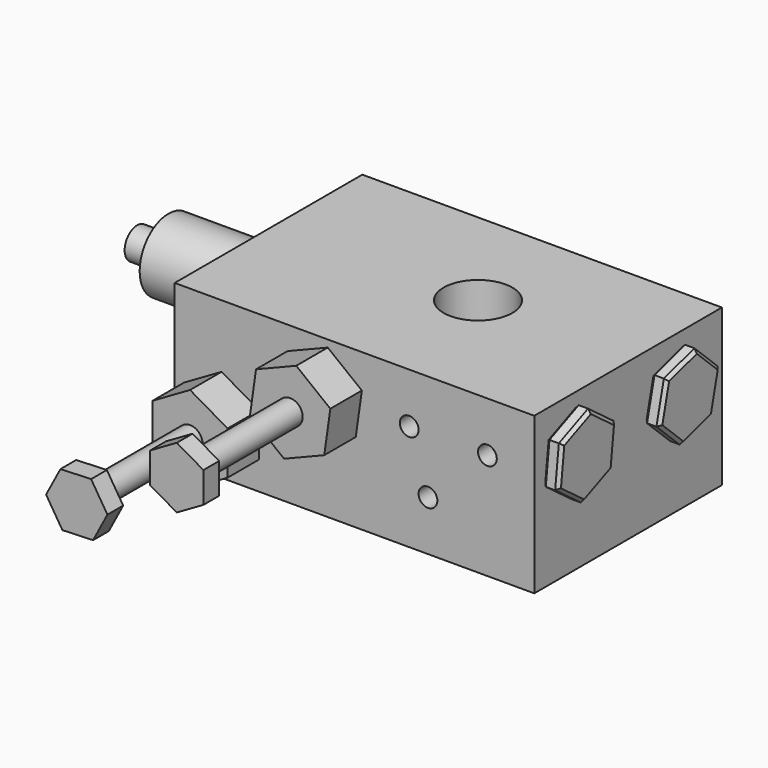
from build123d import *

# Parameters (mm, degrees)
F0_W            = 115
F0_H            = 75
F1_DEPTH        = 50
F3_D            = 5
F3_DEPTH        = 35
F3_TIP          = 1.5021515476
F6_D            = 13
F6_DEPTH        = 27
F6_CBORE_D      = 19
F6_CBORE_DEPTH  = 20
F6_TIP          = 3.9055940237
F8_D            = 6
F8_DEPTH        = 57
F8_TIP          = 1.8025818571
F10_D           = 6
F10_DEPTH       = 83
F10_TIP         = 1.8025818571
F11_D           = 13
F11_DEPTH       = 30
F11_CBORE_D     = 19
F11_CBORE_DEPTH = 22
F11_TIP         = 3.9055940237
F12_D           = 6
F12_DEPTH       = 4
F12_START       = 32.1030122
F12_TIP         = 1.8025818571
F13_D           = 6
F13_DEPTH       = 15
F13_START       = 29.1030122
F13_TIP         = 1.8025818571
F14_D           = 6
F14_DEPTH       = 16
F14_TIP         = 1.8025818571
F15_D           = 6
F15_DEPTH       = 30
F15_START       = 29.1030122
F15_TIP         = 1.8025818571
F16_D           = 6
F16_DEPTH       = 50
F16_TIP         = 1.8025818571
F17_D           = 6
F17_DEPTH       = 34
F17_TIP         = 1.8025818571
F18_D           = 13
F18_DEPTH       = 30
F18_CBORE_D     = 19
F18_CBORE_DEPTH = 22
F18_TIP         = 3.9055940237
F19_D           = 13
F19_DEPTH       = 30
F19_CBORE_D     = 19
F19_CBORE_DEPTH = 22
F19_TIP         = 3.9055940237
F20_D           = 6
F20_DEPTH       = 15
F20_START       = 32.1030122
F20_TIP         = 1.8025818571
F21_D           = 6
F21_DEPTH       = 35
F21_TIP         = 1.8025818571
F22_D           = 6
F22_DEPTH       = 4
F22_START       = 38
F22_TIP         = 1.8025818571
F24_D           = 5
F24_DEPTH       = 15
F24_TIP         = 1.5021515476
F25_D           = 22
F26_R           = 11.5
F27_DEPTH       = 26
F29_D           = 6
F29_DEPTH       = 82
F29_TIP         = 1.8025818571
F30_DEPTH       = 5
F31_SIZE        = 1
F31_2_SIZE      = 1
F28_R           = 5
F32_DEPTH       = 12
F9_R            = 11.5
F33_DEPTH       = 30
F34_R           = 5
F35_DEPTH       = 10
F36_D           = 6
F36_DEPTH       = 18
F36_TIP         = 1.8025818571
F38_DEPTH       = 12.6
F39_R           = 4
F40_DEPTH       = 39
F41_R           = 4
F42_DEPTH       = 6.3
F43_R           = 4
F44_DEPTH       = 39
F45_R           = 4
F46_DEPTH       = 6.3
F47_D           = 5
F47_DEPTH       = 6
F47_TIP         = 1.5021515476


# Not quite as in the source:
# - a feature names something its author has since deleted; it is built from what else it names


with BuildPart() as f1:
    # F0 (on Top) → F1 (new body)
    with BuildSketch(Plane.XY):
        with Locations((-7.5, -2.5)):
            Rectangle(F0_W, F0_H)
    extrude(amount=F1_DEPTH)

    # F3
    with Locations(Plane(origin=(0, 0, 0), x_dir=(1, 0, 0), z_dir=(0, 0, -1))):
        with Locations((-16, -7.32)):
            Hole(F3_D / 2, depth=F3_DEPTH)
            with Locations((0, 0, -(F3_DEPTH + F3_TIP / 2))):  # 118° drill point
                Cone(0, F3_D / 2, F3_TIP, mode=Mode.SUBTRACT)

    # F6
    with Locations(Plane.YZ.offset(50)):
        with Locations((16, 34), (-25, 34)):
            CounterBoreHole(F6_D / 2, F6_CBORE_D / 2, F6_CBORE_DEPTH, depth=F6_DEPTH)
            with Locations((0, 0, -(F6_DEPTH + F6_TIP / 2))):  # 118° drill point
                Cone(0, F6_D / 2, F6_TIP, mode=Mode.SUBTRACT)

    # F8
    with Locations(Plane.XZ.offset(40)):
        with Locations((16, 16)):
            Hole(F8_D / 2, depth=F8_DEPTH)
            with Locations((0, 0, -(F8_DEPTH + F8_TIP / 2))):  # 118° drill point
                Cone(0, F8_D / 2, F8_TIP, mode=Mode.SUBTRACT)

    # F10
    with Locations(Plane(origin=(-65, 0, 0), x_dir=(0, -1, 0), z_dir=(-1, 0, 0))):
        with Locations((25, 16)):
            Hole(F10_D / 2, depth=F10_DEPTH)
            with Locations((0, 0, -(F10_DEPTH + F10_TIP / 2))):  # 118° drill point
                Cone(0, F10_D / 2, F10_TIP, mode=Mode.SUBTRACT)

    # F11
    with Locations(Plane.XZ.offset(40)):
        with Locations((-50, 16), (-18, 34)):
            CounterBoreHole(F11_D / 2, F11_CBORE_D / 2, F11_CBORE_DEPTH, depth=F11_DEPTH)
            with Locations((0, 0, -(F11_DEPTH + F11_TIP / 2))):  # 118° drill point
                Cone(0, F11_D / 2, F11_TIP, mode=Mode.SUBTRACT)

    # F12
    # its depths count from where the whole tool has entered the part; down to there all is cleared
    with Locations(Plane.XZ.offset(40)):
        with Locations((-50, 16)):
            Hole(F12_D / 2, depth=F12_START)
    with Locations(Plane.XZ.offset(40).offset(-F12_START)):
        with Locations((-50, 16)):
            Hole(F12_D / 2, depth=F12_DEPTH)
            with Locations((0, 0, -(F12_DEPTH + F12_TIP / 2))):  # 118° drill point
                Cone(0, F12_D / 2, F12_TIP, mode=Mode.SUBTRACT)

    # F13
    # its depths count from where the whole tool has entered the part; down to there all is cleared
    with Locations(Plane.YZ.offset(50)):
        with Locations((16, 34)):
            Hole(F13_D / 2, depth=F13_START)
    with Locations(Plane.YZ.offset(50).offset(-F13_START)):
        with Locations((16, 34)):
            Hole(F13_D / 2, depth=F13_DEPTH)
            with Locations((0, 0, -(F13_DEPTH + F13_TIP / 2))):  # 118° drill point
                Cone(0, F13_D / 2, F13_TIP, mode=Mode.SUBTRACT)

    # F14
    with Locations(Plane.XZ.offset(40)):
        with Locations((10, 34)):
            Hole(F14_D / 2, depth=F14_DEPTH)
            with Locations((0, 0, -(F14_DEPTH + F14_TIP / 2))):  # 118° drill point
                Cone(0, F14_D / 2, F14_TIP, mode=Mode.SUBTRACT)

    # F15
    # its depths count from where the whole tool has entered the part; down to there all is cleared
    with Locations(Plane.YZ.offset(50).offset(-F15_START)):
        with Locations((-25, 34)):
            Hole(F15_D / 2, depth=F15_DEPTH)
            with Locations((0, 0, -(F15_DEPTH + F15_TIP / 2))):  # 118° drill point
                Cone(0, F15_D / 2, F15_TIP, mode=Mode.SUBTRACT)

    # F16
    with Locations(Plane.XZ.offset(40)):
        with Locations((35, 34)):
            Hole(F16_D / 2, depth=F16_DEPTH)
            with Locations((0, 0, -(F16_DEPTH + F16_TIP / 2))):  # 118° drill point
                Cone(0, F16_D / 2, F16_TIP, mode=Mode.SUBTRACT)

    # F17
    with Locations(Plane(origin=(0, 0, 0), x_dir=(1, 0, 0), z_dir=(0, 0, -1))):
        with Locations((35, 7)):
            Hole(F17_D / 2, depth=F17_DEPTH)
            with Locations((0, 0, -(F17_DEPTH + F17_TIP / 2))):  # 118° drill point
                Cone(0, F17_D / 2, F17_TIP, mode=Mode.SUBTRACT)

    # F18
    with Locations(Plane(origin=(-65, 0, 0), x_dir=(0, -1, 0), z_dir=(-1, 0, 0))):
        with Locations((5, 34)):
            CounterBoreHole(F18_D / 2, F18_CBORE_D / 2, F18_CBORE_DEPTH, depth=F18_DEPTH)
            with Locations((0, 0, -(F18_DEPTH + F18_TIP / 2))):  # 118° drill point
                Cone(0, F18_D / 2, F18_TIP, mode=Mode.SUBTRACT)

    # F19
    with Locations(Plane(origin=(-65, 0, 0), x_dir=(0, -1, 0), z_dir=(-1, 0, 0))):
        with Locations((-16, 16)):
            CounterBoreHole(F19_D / 2, F19_CBORE_D / 2, F19_CBORE_DEPTH, depth=F19_DEPTH)
            with Locations((0, 0, -(F19_DEPTH + F19_TIP / 2))):  # 118° drill point
                Cone(0, F19_D / 2, F19_TIP, mode=Mode.SUBTRACT)

    # F20
    # its depths count from where the whole tool has entered the part; down to there all is cleared
    with Locations(Plane(origin=(-65, 0, 0), x_dir=(0, -1, 0), z_dir=(-1, 0, 0))):
        with Locations((5, 34)):
            Hole(F20_D / 2, depth=F20_START)
    with Locations(Plane(origin=(-65, 0, 0), x_dir=(0, -1, 0), z_dir=(-1, 0, 0)).offset(-F20_START)):
        with Locations((5, 34)):
            Hole(F20_D / 2, depth=F20_DEPTH)
            with Locations((0, 0, -(F20_DEPTH + F20_TIP / 2))):  # 118° drill point
                Cone(0, F20_D / 2, F20_TIP, mode=Mode.SUBTRACT)

    # F21
    with Locations(Plane(origin=(0, 0, 0), x_dir=(1, 0, 0), z_dir=(0, 0, -1))):
        with Locations((-50, 5)):
            Hole(F21_D / 2, depth=F21_DEPTH)
            with Locations((0, 0, -(F21_DEPTH + F21_TIP / 2))):  # 118° drill point
                Cone(0, F21_D / 2, F21_TIP, mode=Mode.SUBTRACT)

    # F22
    # its depths count from where the whole tool has entered the part; down to there all is cleared
    with Locations(Plane.XZ.offset(40)):
        with Locations((-18, 34)):
            Hole(F22_D / 2, depth=F22_START)
    with Locations(Plane.XZ.offset(40).offset(-F22_START)):
        with Locations((-18, 34)):
            Hole(F22_D / 2, depth=F22_DEPTH)
            with Locations((0, 0, -(F22_DEPTH + F22_TIP / 2))):  # 118° drill point
                Cone(0, F22_D / 2, F22_TIP, mode=Mode.SUBTRACT)

    # F24
    with Locations(Plane(origin=(0, 35, 0), x_dir=(-1, 0, 0), z_dir=(0, 1, 0))):
        with Locations((35, 25), (-25, 25)):
            Hole(F24_D / 2, depth=F24_DEPTH)
            with Locations((0, 0, -(F24_DEPTH + F24_TIP / 2))):  # 118° drill point
                Cone(0, F24_D / 2, F24_TIP, mode=Mode.SUBTRACT)

    # F25 (through all)
    with Locations(Plane(origin=(0, 0, 0), x_dir=(1, 0, 0), z_dir=(0, 0, -1))):
        with Locations((0, 0)):
            Hole(F25_D / 2)

    # F29
    with Locations(Plane(origin=(-65, 0, 0), x_dir=(0, -1, 0), z_dir=(-1, 0, 0))):
        with Locations((-16, 16)):
            Hole(F29_D / 2, depth=F29_DEPTH)
            with Locations((0, 0, -(F29_DEPTH + F29_TIP / 2))):  # 118° drill point
                Cone(0, F29_D / 2, F29_TIP, mode=Mode.SUBTRACT)

    # F36
    with Locations(Plane(origin=(0, 0, 0), x_dir=(1, 0, 0), z_dir=(0, 0, -1))):
        with Locations((-50, -16)):
            Hole(F36_D / 2, depth=F36_DEPTH)
            with Locations((0, 0, -(F36_DEPTH + F36_TIP / 2))):  # 118° drill point
                Cone(0, F36_D / 2, F36_TIP, mode=Mode.SUBTRACT)

    # F47
    with Locations(Plane(origin=(0, 0, 0), x_dir=(1, 0, 0), z_dir=(0, 0, -1))):
        with Locations((16, -22.32), (-16, 7.68)):
            Hole(F47_D / 2, depth=F47_DEPTH)
            with Locations((0, 0, -(F47_DEPTH + F47_TIP / 2))):  # 118° drill point
                Cone(0, F47_D / 2, F47_TIP, mode=Mode.SUBTRACT)


with BuildPart() as f27:
    # F26 (on face) → F27 (new body)
    with BuildSketch(Plane(origin=(-65, 0, 0), x_dir=(0, -1, 0), z_dir=(-1, 0, 0))):
        with Locations((-16, 16)):
            Circle(F26_R)
    extrude(amount=F27_DEPTH)

    # F28 (on face) → F32 (join)
    with BuildSketch(Plane(origin=(-91, 0, 0), x_dir=(0, -1, 0), z_dir=(-1, 0, 0))):
        with Locations((-16, 16)):
            Circle(F28_R)
    extrude(amount=F32_DEPTH)


with BuildPart() as f30:
    # F5 (on face) → F30 (new body)
    with BuildSketch(Plane.YZ.offset(50)):
        Polygon((-23.5270221617, 46.6160084663), (-35.189294907, 41.5836404603), (-36.6622727453, 28.967631994), (-26.4729778383, 21.3839915337), (-14.810705093, 26.4163595397), (-13.3377272547, 39.032368006), align=None)
    extrude(amount=F30_DEPTH)

    # F31
    f31_edges = [f30.edges().sort_by_distance(p)[0] for p in [
        (50, -20.641841, 23.900176),
        (50, -31.567625, 25.175812),
        (50, -35.925784, 35.275636),
        (55, -31.567625, 25.175812),
        (55, -20.641841, 23.900176),
        (55, -14.074216, 32.724364),
        (55, -18.432375, 42.824188),
        (55, -29.358159, 44.099824),
        (55, -35.925784, 35.275636),
        (50, -29.358159, 44.099824),
        (50, -18.432375, 42.824188),
        (50, -14.074216, 32.724364),
    ]]
    chamfer(f31_edges, length=F31_SIZE)


with BuildPart() as f30b:
    # F5 (on face) → F30, piece 2 (new body)
    with BuildSketch(Plane.YZ.offset(50)):
        Polygon((18.9808178574, 46.3469857955), (6.7976055696, 42.7549568863), (3.8167877122, 30.4079710908), (13.0191821426, 21.6530142045), (25.2023944304, 25.2450431137), (28.1832122878, 37.5920289092), align=None)
    extrude(amount=F30_DEPTH)

    # F31#2
    f31_2_edges = [f30b.edges().sort_by_distance(p)[0] for p in [
        (55, 8.417985, 26.030493),
        (50, 8.417985, 26.030493),
        (55, 19.110788, 23.449029),
        (50, 19.110788, 23.449029),
        (55, 26.692803, 31.418536),
        (50, 26.692803, 31.418536),
        (55, 23.582015, 41.969507),
        (50, 23.582015, 41.969507),
        (55, 5.307197, 36.581464),
        (50, 5.307197, 36.581464),
        (50, 12.889212, 44.550971),
        (55, 12.889212, 44.550971),
    ]]
    chamfer(f31_2_edges, length=F31_2_SIZE)


with BuildPart() as f33:
    # F9 (on face) → F33 (new body)
    with BuildSketch(Plane(origin=(-65, 0, 0), x_dir=(0, -1, 0), z_dir=(-1, 0, 0))):
        with Locations((5, 34)):
            Circle(F9_R)
    extrude(amount=F33_DEPTH)

    # F34 (on face) → F35 (join)
    with BuildSketch(Plane(origin=(-95, 0, 0), x_dir=(0, -1, 0), z_dir=(-1, 0, 0))):
        with Locations((5, 34)):
            Circle(F34_R)
    extrude(amount=F35_DEPTH)


with BuildPart() as f38:
    # F37 (on face) → F38 (new body)
    with BuildSketch(Plane.XZ.offset(40)):
        Polygon((-38, 9.0717967697), (-38, 22.9282032303), (-50, 29.8564064606), (-62, 22.9282032303), (-62, 9.0717967697), (-50, 2.1435935394), align=None)
    extrude(amount=F38_DEPTH)

    # F39 (on face) → F40 (join)
    with BuildSketch(Plane.XZ.offset(52.6)):
        with Locations((-50, 16)):
            Circle(F39_R)
    extrude(amount=F40_DEPTH)

    # F41 (on face) → F42 (join)
    with BuildSketch(Plane.XZ.offset(91.6)):
        Polygon((-40.1919154978, 16.3671671712), (-45.4139338466, 24.6776339269), (-55.2220183487, 24.3104667558), (-59.8080845022, 15.6328328288), (-54.5860661534, 7.3223660731), (-44.7779816513, 7.6895332442), align=None)
        with Locations((-50, 16)):
            Circle(F41_R, mode=Mode.SUBTRACT)
        with Locations((-50, 16)):
            Circle(F41_R)
    extrude(amount=F42_DEPTH)


with BuildPart() as f38b:
    # F37 (on face) → F38, piece 2 (new body)
    with BuildSketch(Plane.XZ.offset(40)):
        Polygon((-7.0902049982, 25.4573790311), (-5.1469757251, 39.1768491372), (-16.056770727, 47.7194701061), (-28.9097950018, 42.5426209689), (-30.8530242749, 28.8231508628), (-19.943229273, 20.2805298939), align=None)
    extrude(amount=F38_DEPTH)

    # F43 (on face) → F44 (join)
    with BuildSketch(Plane.XZ.offset(52.6)):
        with Locations((-18, 34)):
            Circle(F43_R)
    extrude(amount=F44_DEPTH)

    # F45 (on face) → F46 (join)
    with BuildSketch(Plane.XZ.offset(91.6)):
        Polygon((-9.5, 29.0925227119), (-9.5, 38.9074772881), (-18, 43.8149545762), (-26.5, 38.9074772881), (-26.5, 29.0925227119), (-18, 24.1850454238), align=None)
        with Locations((-18, 34)):
            Circle(F45_R, mode=Mode.SUBTRACT)
        with Locations((-18, 34)):
            Circle(F45_R)
    extrude(amount=F46_DEPTH)


solid = Compound([f1.part, f27.part, f30.part, f30b.part, f33.part, f38.part, f38b.part])
